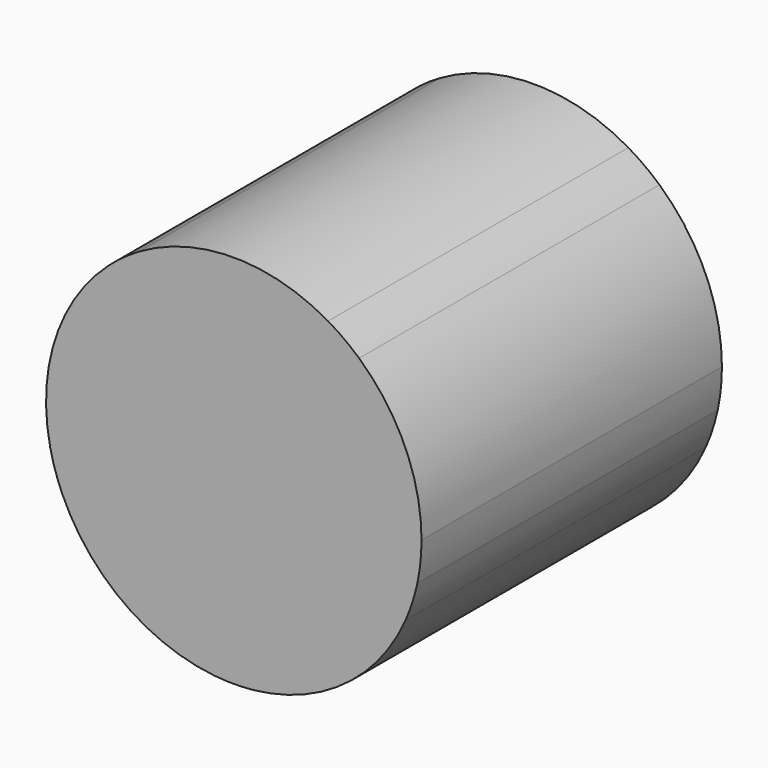
from build123d import *

# Parameters (mm, degrees)
F1_DEPTH = 50.8


with BuildPart() as f1:
    # F0 (on Front) → F1 (new body)
    with BuildSketch(Plane.XZ):
        with BuildLine():
            ThreePointArc((24.8326570204, -5.338459076), (25.2577660168, -2.6842607624), (25.4, 0))
            ThreePointArc((25.4, 0), (23.1920807644, 10.3579626287), (16.9521740302, 18.9151736881))
            ThreePointArc((16.9521740302, 18.9151736881), (14.9297454082, 20.5490316571), (12.750889326, 21.9675856979))
            ThreePointArc((12.750889326, 21.9675856979), (0, 25.4), (-12.750889326, 21.9675856979))
            ThreePointArc((-12.750889326, 21.9675856979), (-14.9297454082, 20.5490316571), (-16.9521740302, 18.9151736881))
            ThreePointArc((-16.9521740302, 18.9151736881), (-24.1568355139, 7.8490316571), (-24.8326570204, -5.338459076))
            ThreePointArc((-24.8326570204, -5.338459076), (-24.1568355139, -7.8490316571), (-23.2279090598, -10.2773654556))
            ThreePointArc((-23.2279090598, -10.2773654556), (-14.9297454082, -20.5490316571), (-2.5965367436, -25.2669348545))
            ThreePointArc((-2.5965367436, -25.2669348545), (0, -25.4), (2.5965367436, -25.2669348545))
            ThreePointArc((2.5965367436, -25.2669348545), (14.9297454082, -20.5490316571), (23.2279090598, -10.2773654556))
            ThreePointArc((23.2279090598, -10.2773654556), (24.1568355139, -7.8490316571), (24.8326570204, -5.338459076))
        make_face()
    extrude(amount=F1_DEPTH)


solid = f1.part
